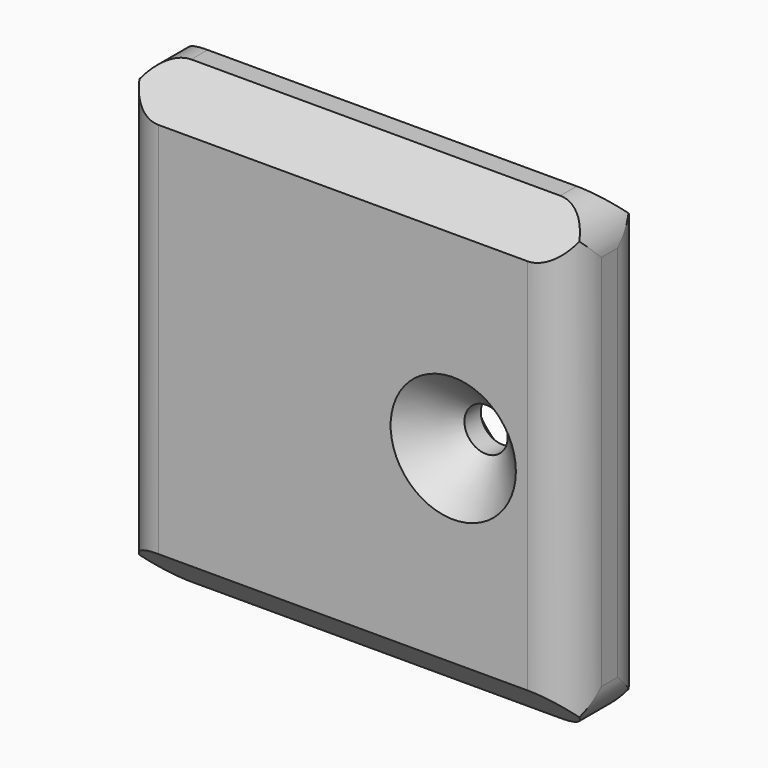
from build123d import *

# Parameters (mm, degrees)
F0_W        = 55.88
F0_H        = 56.9722
F0_R        = 2.6797
F1_DEPTH    = 6.35
F2_R        = 5.08
F3_R        = 5.08
F4_T1_DEPTH = 71.8482991577
F5_T1_DEPTH = 71.8482991577


# Not quite as in the source:
# - a fillet or chamfer that OpenCascade refuses, or shapes differently, is made with other operations: its cross-section is extruded or revolved along the edge and cut away or added


with BuildPart() as f1:
    # F0 (on Front) → F1 (new body, symmetric)
    with BuildSketch(Plane.XZ):
        Rectangle(F0_W, F0_H)
        with Locations((13.660245575, 0)):
            Circle(F0_R, mode=Mode.SUBTRACT)
    extrude(amount=F1_DEPTH, both=True)

    # F2
    f2_edges = [f1.edges().sort_by_distance(p)[0] for p in [
        (-27.94, 6.35, 0),
        (-27.94, 0, -28.4861),
        (-27.94, -6.35, 0),
        (-27.94, 0, 28.4861),
    ]]
    fillet(f2_edges, radius=F2_R)

    # F3
    f3_edges = [f1.edges().sort_by_distance(p)[0] for p in [
        (27.94, 0, -28.4861),
        (27.94, 6.35, 0),
        (27.94, 0, 28.4861),
        (27.94, -6.35, 0),
    ]]
    fillet(f3_edges, radius=F3_R)

    # F4: chamfer of 5.08 on 5 edges, made by hand

    # F4_s2 → F4_t1 (cut)
    with BuildSketch(Plane.YZ.offset(-35.9241495789)):
        Polygon((-1.27, -28.4861), (-6.35, -23.4061), (-6.35, -28.4861), align=None)
        Polygon((-6.35, 23.4061), (-1.27, 28.4861), (-6.35, 28.4861), align=None)
    extrude(amount=F4_T1_DEPTH, mode=Mode.SUBTRACT)

    # F4_s3 → F4_t4 (revolve, cut)
    with BuildSketch(Plane.XY):
        Polygon((21.419945575, -6.35), (16.339945575, -1.27), (16.339945575, -6.35), align=None)
    revolve(axis=Axis((13.660245575, -6.35, 0), (0, -1, 0)), mode=Mode.SUBTRACT)

    # F5: chamfer of 5.08 on 5 edges, made by hand

    # F5_s2 → F5_t1 (cut)
    with BuildSketch(Plane.YZ.offset(-35.9241495789)):
        Polygon((1.27, -28.4861), (6.35, -23.4061), (6.35, -28.4861), align=None)
        Polygon((6.35, 23.4061), (1.27, 28.4861), (6.35, 28.4861), align=None)
    extrude(amount=F5_T1_DEPTH, mode=Mode.SUBTRACT)

    # F5_s3 → F5_t4 (revolve, cut)
    with BuildSketch(Plane.XY):
        Polygon((21.419945575, 6.35), (16.339945575, 1.27), (16.339945575, 6.35), align=None)
    revolve(axis=Axis((13.660245575, 6.35, 0), (0, -1, 0)), mode=Mode.SUBTRACT)


solid = f1.part
